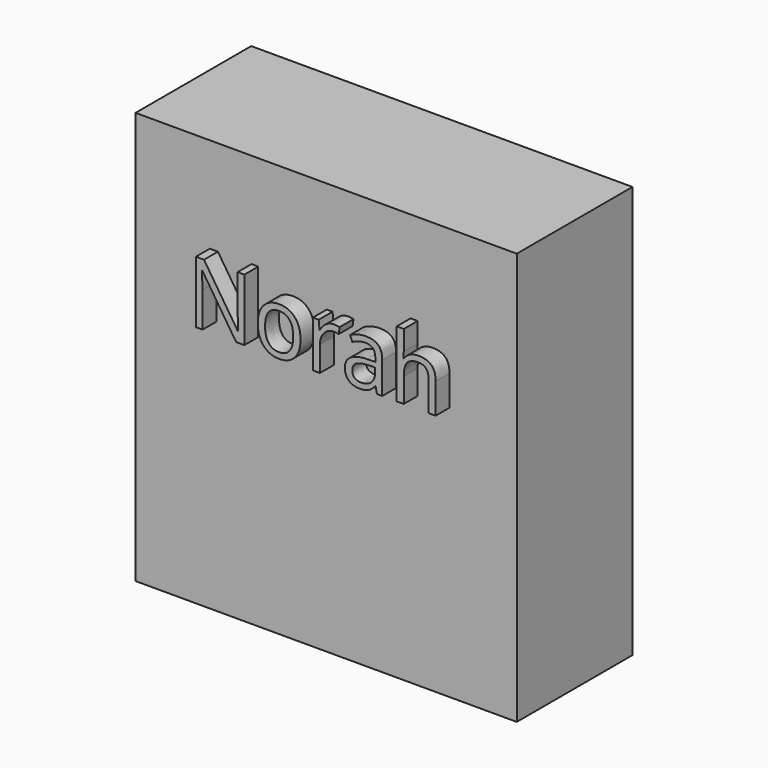
from build123d import *

# Parameters (mm, degrees)
F0_W         = 66.9851116836
F0_H         = 72.4240802228
F1_DEPTH     = 25.4
F2_T         = -2.54
F3_TEXT_SIZE = 15.2734612736
F4_DEPTH     = 28.448


# Not quite as in the source:
# - Text() gives the source's letters only with a copy of the font that has no kerning and outlines rounded to 1/6400 em; it was checked with that copy


with BuildPart() as f1:
    # F0 (on Front) → F1 (new body)
    with BuildSketch(Plane.XZ):
        with Locations((0.4293899983, 4.7233086079)):
            Rectangle(F0_W, F0_H)
    extrude(amount=F1_DEPTH)

    # F2
    f2_openings = [f1.faces().sort_by_distance(p)[0] for p in [
        (0.42939, -12.7, -31.488732),
    ]]
    offset(amount=F2_T, openings=f2_openings)

    # F3 (on Front) → F4 (join)
    with BuildSketch(Plane.XZ):
        with Locations((-21.5216809884, 13.2616581395)):
            Text('Norah', F3_TEXT_SIZE, font='Open Sans', text_align=(TextAlign.LEFT, TextAlign.BOTTOM))
    extrude(amount=F4_DEPTH)


solid = f1.part
